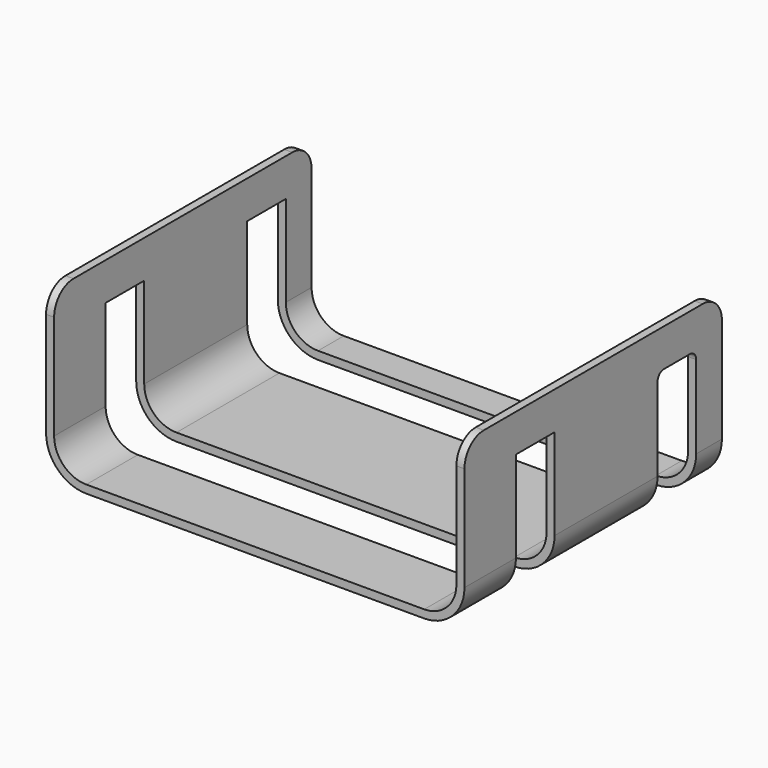
from build123d import *

# Parameters (mm, degrees)
F2_DEPTH = 200
F3_W     = 30
F3_H     = 100
F4_DEPTH = 500
F6_R     = 15
F7_R     = 5


with BuildPart() as f2:
    # F0 (on Front) → F2 (new body)
    with BuildSketch(Plane.XZ):
        with BuildLine():
            Line((-127.5536519289, -36.5021181107), (-127.5536519289, 43.4978818893))
            Line((-127.5536519289, 43.4978818893), (-132.5536519289, 43.4978818893))
            Line((-132.5536519289, 43.4978818893), (-132.5536519289, -36.5021181107))
            ThreePointArc((-132.5536519289, -36.5021181107), (-125.2313214586, -54.1797876403), (-107.5536519289, -61.5021181107))
            Line((-107.5536519289, -61.5021181107), (102.4463480711, -61.5021181107))
            ThreePointArc((102.4463480711, -61.5021181107), (120.1240176008, -54.1797876403), (127.4463480711, -36.5021181107))
            Line((127.4463480711, -36.5021181107), (127.4463480711, 43.4978818893))
            Line((127.4463480711, 43.4978818893), (122.4463480711, 43.4978818893))
            Line((122.4463480711, 43.4978818893), (122.4463480711, -36.5021181107))
            ThreePointArc((122.4463480711, -36.5021181107), (116.5884836948, -50.6442537344), (102.4463480711, -56.5021181107))
            Line((102.4463480711, -56.5021181107), (-107.5536519289, -56.5021181107))
            ThreePointArc((-107.5536519289, -56.5021181107), (-121.6957875526, -50.6442537344), (-127.5536519289, -36.5021181107))
        make_face()
    extrude(amount=F2_DEPTH)


with BuildPart() as f4:
    # F3 (on offset) → F4 (new body)
    with BuildSketch(Plane.YZ.offset(200)):
        with Locations((-145, -29.9103426556)):
            Rectangle(F3_W, F3_H)
    extrude(amount=-F4_DEPTH)


with BuildPart() as f4b:
    # F3 (on offset) → F4, piece 2 (new body)
    with BuildSketch(Plane.YZ.offset(200)):
        with Locations((-35, -29.9103426556)):
            Rectangle(F3_W, F3_H)
    extrude(amount=-F4_DEPTH)


with BuildPart() as f2_1:
    add(f2.part)

    # F5: cut F4, F4b
    add(f4.part, mode=Mode.SUBTRACT)
    add(f4b.part, mode=Mode.SUBTRACT)

    # F6
    f6_edges = [f2_1.edges().sort_by_distance(p)[0] for p in [
        (-130.053652, -200, 43.497882),
        (-130.053652, 0, 43.497882),
        (124.946348, -200, 43.497882),
        (124.946348, 0, 43.497882),
    ]]
    fillet(f6_edges, radius=F6_R)

    # F7
    f7_edges = [f2_1.edges().sort_by_distance(p)[0] for p in [
        (124.946348, -20, 20.089657),
        (124.946348, -50, 20.089657),
    ]]
    fillet(f7_edges, radius=F7_R)


solid = f2_1.part
